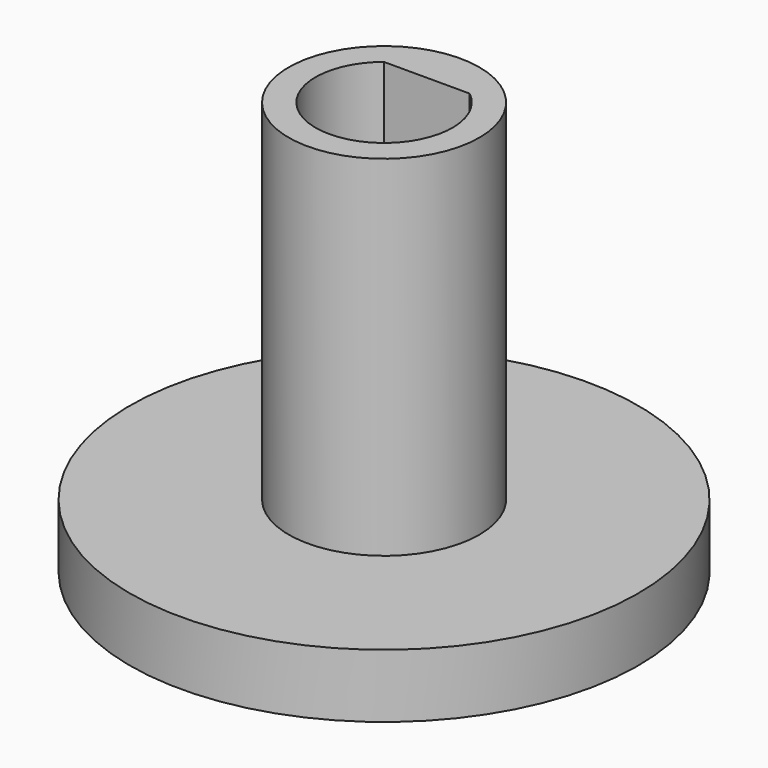
from build123d import *

# Parameters (mm, degrees)
F0_R     = 12.7
F1_DEPTH = 3.175
F2_R     = 4.7625
F3_DEPTH = 17.4625
F4_DEPTH = 25.4


# Not quite as in the source:
# - a length typed as a fraction of an inch, garbled in the dataset ("3 / 203.2 mm" for 3/8 in), is restored


with BuildPart() as f1:
    # F0 (on Top) → F1 (new body)
    with BuildSketch(Plane.XY):
        Circle(F0_R)
        with BuildLine():
            ThreePointArc((2.1403987868, 2.67081), (0, -3.42265), (-2.1403987868, 2.67081))
            Line((-2.1403987868, 2.67081), (2.1403987868, 2.67081))
        make_face(mode=Mode.SUBTRACT)
    extrude(amount=F1_DEPTH)

    # F2 (on face) → F3 (join)
    with BuildSketch(Plane.XY.offset(3.175)):
        Circle(F2_R)
        with BuildLine():
            Line((-2.1403987868, 2.67081), (2.1403987868, 2.67081))
            ThreePointArc((2.1403987868, 2.67081), (0, -3.42265), (-2.1403987868, 2.67081))
        make_face(mode=Mode.SUBTRACT)
    extrude(amount=F3_DEPTH)

    # F2 (on face) → F4 (cut)
    with BuildSketch(Plane.XY.offset(3.175)):
        with BuildLine():
            ThreePointArc((-4.8118133156, 7.58825), (-3.6688133156, 8.73125), (-4.8118133156, 9.87425))
            Line((-4.8118133156, 9.87425), (-7.9868133156, 9.87425))
            ThreePointArc((-7.9868133156, 9.87425), (-9.1568912319, 8.8000763046), (-10.1837351663, 7.58825))
            Line((-10.1837351663, 7.58825), (-4.8118133156, 7.58825))
        make_face()
    extrude(amount=-F4_DEPTH, mode=Mode.SUBTRACT)


solid = f1.part
